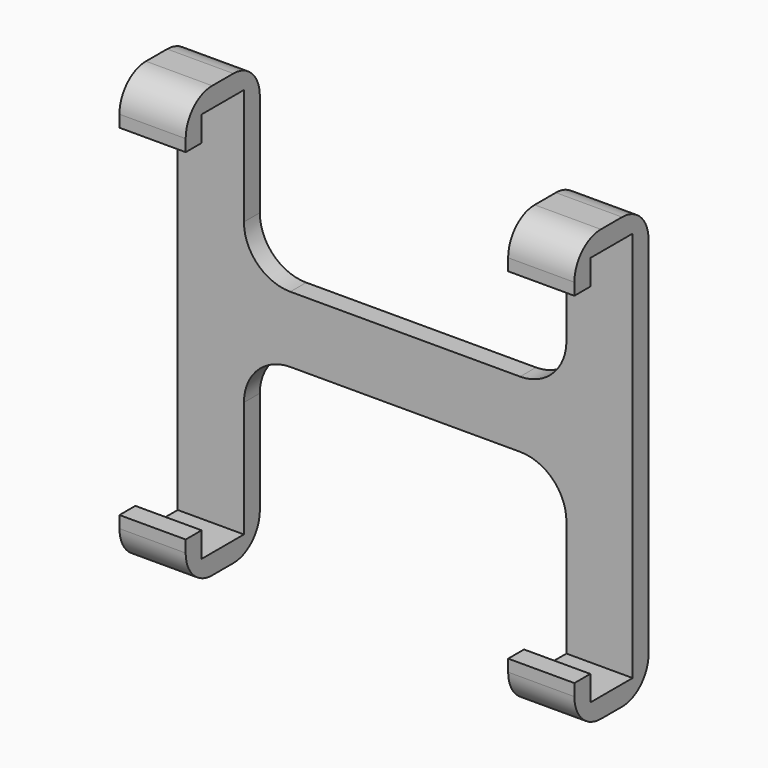
from build123d import *

# Parameters (mm, degrees)
F1_DEPTH      = 43.6245
F1_DEPTH_BACK = 43.6245
F2_R          = 1.905
F3_DEPTH      = 2.794
F5_DEPTH      = 25.4


# Not quite as in the source:
# - a length typed as a fraction of an inch, garbled in the dataset ("3 / 203.2 mm" for 3/8 in), is restored


with BuildPart() as f1:
    # F0 (on Right) → F1 (new body, two sides)
    with BuildSketch(Plane.YZ) as f1_sk:
        with BuildLine():
            Line((-8.008403407, 37.52215), (-8.008403407, 0))
            Line((-8.008403407, 0), (-8.008403407, -37.52215))
            Line((-8.008403407, -37.52215), (-18.168403407, -37.52215))
            Line((-18.168403407, -37.52215), (-18.168403407, -32.69615))
            Line((-18.168403407, -32.69615), (-21.978403407, -32.69615))
            Line((-21.978403407, -32.69615), (-21.978403407, -34.98215))
            ThreePointArc((-21.978403407, -34.98215), (-20.1185314675, -39.4722780605), (-15.628403407, -41.33215))
            Line((-15.628403407, -41.33215), (-10.548403407, -41.33215))
            ThreePointArc((-10.548403407, -41.33215), (-6.0582753465, -39.4722780605), (-4.198403407, -34.98215))
            Line((-4.198403407, -34.98215), (-4.198403407, 0))
            Line((-4.198403407, 0), (-4.198403407, 34.98215))
            ThreePointArc((-4.198403407, 34.98215), (-6.0582753465, 39.4722780605), (-10.548403407, 41.33215))
            Line((-10.548403407, 41.33215), (-15.628403407, 41.33215))
            ThreePointArc((-15.628403407, 41.33215), (-20.1185314675, 39.4722780605), (-21.978403407, 34.98215))
            Line((-21.978403407, 34.98215), (-21.978403407, 32.69615))
            Line((-21.978403407, 32.69615), (-18.168403407, 32.69615))
            Line((-18.168403407, 32.69615), (-18.168403407, 37.52215))
            Line((-18.168403407, 37.52215), (-8.008403407, 37.52215))
        make_face()
    extrude(amount=F1_DEPTH)
    extrude(f1_sk.sketch, amount=-F1_DEPTH_BACK)

    # F2 (on face) → F3 (cut)
    with BuildSketch(Plane(origin=(0, -4.198403407, 0), x_dir=(-1, 0, 0), z_dir=(0, 1, 0))):
        Circle(F2_R)
    extrude(amount=-F3_DEPTH, mode=Mode.SUBTRACT)

    # F4 (on face) → F5 (cut)
    with BuildSketch(Plane(origin=(0, -4.198403407, 0), x_dir=(-1, 0, 0), z_dir=(0, 1, 0))):
        with BuildLine():
            Line((-22.0345, 6.35), (22.0345, 6.35))
            ThreePointArc((22.0345, 6.35), (28.3206792847, 8.9538207153), (30.9245, 15.24))
            Line((30.9245, 15.24), (30.9245, 50.7227726401))
            Line((30.9245, 50.7227726401), (-30.9245, 50.7227726401))
            Line((-30.9245, 50.7227726401), (-30.9245, 15.24))
            ThreePointArc((-30.9245, 15.24), (-28.3206792847, 8.9538207153), (-22.0345, 6.35))
        make_face()
        with BuildLine():
            ThreePointArc((30.9245, -15.24), (28.3206792847, -8.9538207153), (22.0345, -6.35))
            Line((22.0345, -6.35), (-22.0345, -6.35))
            ThreePointArc((-22.0345, -6.35), (-28.3206792847, -8.9538207153), (-30.9245, -15.24))
            Line((-30.9245, -15.24), (-30.9245, -50.7227726401))
            Line((-30.9245, -50.7227726401), (30.9245, -50.7227726401))
            Line((30.9245, -50.7227726401), (30.9245, -15.24))
        make_face()
    extrude(amount=-F5_DEPTH, mode=Mode.SUBTRACT)


solid = f1.part
